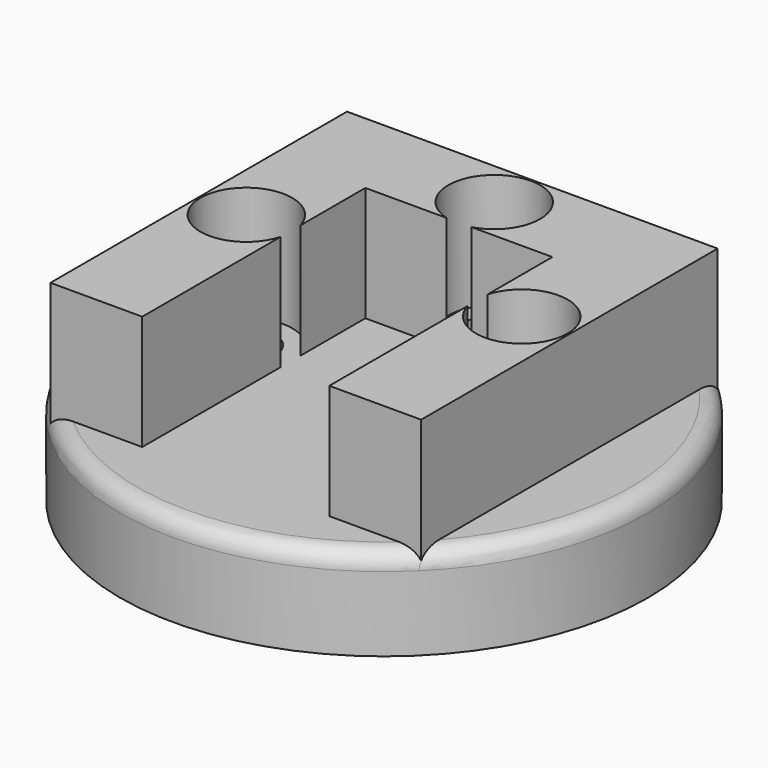
from build123d import *

# Parameters (mm, degrees)
F0_R     = 11.5
F0_R_2   = 1.25
F0_R_3   = 1.5
F1_DEPTH = 4
F3_DEPTH = 5
F5_R     = 2.5
F5_R_2   = 1.5
F6_DEPTH = 2.5


# Not quite as in the source:
# - a fillet or chamfer that OpenCascade refuses, or shapes differently, is made with other operations: its cross-section is extruded or revolved along the edge and cut away or added
# - a feature names something its author has since deleted; it is built from what else it names


with BuildPart() as f1:
    # F0 (on Top) → F1 (new body)
    with BuildSketch(Plane.XY):
        Circle(F0_R)
        with Locations((-6, 0)):
            Circle(F0_R_2, mode=Mode.SUBTRACT)
        Circle(F0_R_3, mode=Mode.SUBTRACT)
        with Locations((6, 0)):
            Circle(F0_R_2, mode=Mode.SUBTRACT)
        with Locations((0, 6)):
            Circle(F0_R_2, mode=Mode.SUBTRACT)
    extrude(amount=F1_DEPTH)

    # F2 (on face) → F3 (join)
    with BuildSketch(Plane.XY.offset(4)):
        with BuildLine():
            Line((0.5425633604, 4.075), (4.075, 4.075))
            Line((4.075, 4.075), (4.075, 0.5425633604))
            ThreePointArc((4.075, 0.5425633604), (6.2738612788, 1.9811612756), (8, 0))
            ThreePointArc((8, 0), (6.2738612788, -1.9811612756), (4.075, -0.5425633604))
            Line((4.075, -0.5425633604), (4.075, -4.075))
            Line((4.075, -4.075), (4.075, -8.075))
            Line((4.075, -8.075), (8.075, -8.075))
            Line((8.075, -8.075), (8.075, 8.075))
            Line((8.075, 8.075), (-8.075, 8.075))
            Line((-8.075, 8.075), (-8.075, -8.075))
            Line((-8.075, -8.075), (-4.075, -8.075))
            Line((-4.075, -8.075), (-4.075, -4.075))
            Line((-4.075, -4.075), (-4.075, -0.5425633604))
            ThreePointArc((-4.075, -0.5425633604), (-8, 0), (-4.075, 0.5425633604))
            Line((-4.075, 0.5425633604), (-4.075, 4.075))
            Line((-4.075, 4.075), (-0.5425633604, 4.075))
            ThreePointArc((-0.5425633604, 4.075), (-1.2072434053, 7.5945417399), (2, 6))
            ThreePointArc((2, 6), (1.5945417399, 4.7927565947), (0.5425633604, 4.075))
        make_face()
    extrude(amount=F3_DEPTH)

    # F4: fillet of radius 0.75 on 1 edges, made by hand


with BuildPart() as f4_tool2:
    # F4_s3 → F4_t4 (revolve)
    with BuildSketch(Plane.XZ):
        with BuildLine():
            ThreePointArc((11.5, 3.25), (11.2803300859, 3.7803300859), (10.75, 4))
            Line((10.75, 4), (11.5, 4))
            Line((11.5, 4), (11.5, 3.25))
        make_face()
    revolve(axis=Axis((0, 0, 4), (0, 0, 1)))

    split(bisect_by=Plane.YZ.offset(8.075), keep=Keep.TOP)


with BuildPart() as f1_1:
    add(f1.part)

    # F4_t1: cut F4_tool2
    add(f4_tool2.part, mode=Mode.SUBTRACT)


with BuildPart() as f4_tool7:
    # F4_s8 → F4_t9 (revolve)
    with BuildSketch(Plane.XZ):
        with BuildLine():
            ThreePointArc((11.5, 3.25), (11.2803300859, 3.7803300859), (10.75, 4))
            Line((10.75, 4), (11.5, 4))
            Line((11.5, 4), (11.5, 3.25))
        make_face()
    revolve(axis=Axis((0, 0, 4), (0, 0, 1)))

    split(bisect_by=Plane.XZ.offset(-8.075), keep=Keep.BOTTOM)


with BuildPart() as f1_2:
    add(f1_1.part)

    # F4_t6: cut F4_tool7
    add(f4_tool7.part, mode=Mode.SUBTRACT)


with BuildPart() as f4_tool12:
    # F4_s13 → F4_t14 (revolve)
    with BuildSketch(Plane.XZ):
        with BuildLine():
            ThreePointArc((11.5, 3.25), (11.2803300859, 3.7803300859), (10.75, 4))
            Line((10.75, 4), (11.5, 4))
            Line((11.5, 4), (11.5, 3.25))
        make_face()
    revolve(axis=Axis((0, 0, 4), (0, 0, 1)))

    split(bisect_by=Plane.XZ.offset(8.075), keep=Keep.TOP)


with BuildPart() as f1_3:
    add(f1_2.part)

    # F4_t11: cut F4_tool12
    add(f4_tool12.part, mode=Mode.SUBTRACT)


with BuildPart() as f4_tool17:
    # F4_s18 → F4_t19 (revolve)
    with BuildSketch(Plane.XZ):
        with BuildLine():
            ThreePointArc((11.5, 3.25), (11.2803300859, 3.7803300859), (10.75, 4))
            Line((10.75, 4), (11.5, 4))
            Line((11.5, 4), (11.5, 3.25))
        make_face()
    revolve(axis=Axis((0, 0, 4), (0, 0, 1)))

    split(bisect_by=Plane.YZ.offset(-8.075), keep=Keep.BOTTOM)


with BuildPart() as f1_4:
    add(f1_3.part)

    # F4_t16: cut F4_tool17
    add(f4_tool17.part, mode=Mode.SUBTRACT)

    # F5 (on face) → F6 (cut)
    with BuildSketch(Plane.XY):
        Circle(F5_R)
        Circle(F5_R_2, mode=Mode.SUBTRACT)
    extrude(amount=F6_DEPTH, mode=Mode.SUBTRACT)


solid = f1_4.part
